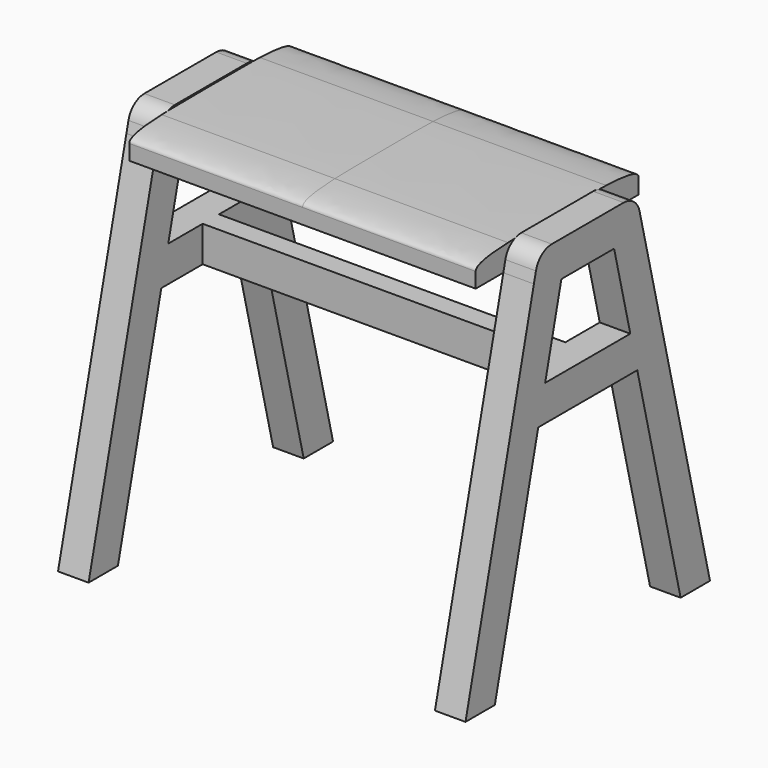
from build123d import *

# Parameters (mm, degrees)
F0_W        = 1
F0_H        = 3.5
F1_DEPTH    = 3
F2_DEPTH    = 20
F4_DEPTH    = 17
F6_T1_DEPTH = 6.9276237231
F6_T3_DEPTH = 6.9276237231


# Not quite as in the source:
# - a fillet or chamfer that OpenCascade refuses, or shapes differently, is made with other operations: its cross-section is extruded or revolved along the edge and cut away or added


with BuildPart() as f1:
    # F0 (on Right) → F1 (new body)
    with BuildSketch(Plane.YZ):
        Polygon((-185.4956659779, 34.4343371689), (-193.88920142, 0), (-190.2867229659, 0), (-184.9662980764, 21.8269531103), (-184.1131562284, 25.3269531103), (-182.1236807397, 33.4887426496), (-178.88920142, 33.4887426496), (-175.6547221004, 33.4887426496), (-173.6652466117, 25.3269531103), (-172.8121047636, 21.8269531103), (-167.4916798742, 0), (-163.88920142, 0), (-172.2827368621, 34.4343371689), (-178.88920142, 34.4343371689), align=None)
        Polygon((-184.8730173458, 36.9887426496), (-185.4956659779, 34.4343371689), (-178.88920142, 34.4343371689), (-172.2827368621, 34.4343371689), (-172.9053854942, 36.9887426496), (-178.88920142, 36.9887426496), align=None)
        Polygon((-184.1131562284, 25.3269531103), (-184.9662980764, 21.8269531103), (-179.88920142, 21.8269531103), (-179.88920142, 25.3269531103), align=None)
        with Locations((-178.38920142, 23.5769531103)):
            Rectangle(F0_W, F0_H)
        with Locations((-179.38920142, 23.5769531103)):
            Rectangle(F0_W, F0_H)
        Polygon((-177.88920142, 21.8269531103), (-172.8121047636, 21.8269531103), (-173.6652466117, 25.3269531103), (-177.88920142, 25.3269531103), align=None)
    extrude(amount=-F1_DEPTH)

    # F0 (on Right) → F2 (join)
    with BuildSketch(Plane.YZ):
        with Locations((-179.38920142, 23.5769531103)):
            Rectangle(F0_W, F0_H)
        with Locations((-178.38920142, 23.5769531103)):
            Rectangle(F0_W, F0_H)
    extrude(amount=-F2_DEPTH)

    # F3 (on face) → F4 (join, through all)
    with BuildSketch(Plane(origin=(-3, 0, 0), x_dir=(0, -1, 0), z_dir=(-1, 0, 0))):
        with BuildLine():
            Line((168.88920142, 34.4301523733), (172.2817167981, 34.4301523733))
            Line((172.2817167981, 34.4301523733), (172.8685340256, 36.8375601227))
            add(Edge.make_bspline(
                [(168.88920142, 35.9301523733), (168.88920142, 36.5362981599), (170.5285389627, 36.7602466997), (172.8685340256, 36.8375601227)],
                knots=[0, 0, 0, 0, 0.2862985804, 0.2862985804, 0.2862985804, 0.2862985804], degree=3))
            Line((168.88920142, 35.9301523733), (168.88920142, 34.4301523733))
        make_face()
        with BuildLine():
            Line((184.9191853663, 36.7993391266), (185.496686042, 34.4301523733))
            Line((185.496686042, 34.4301523733), (188.88920142, 34.4301523733))
            Line((188.88920142, 34.4301523733), (188.88920142, 35.9301523733))
            add(Edge.make_bspline(
                [(184.9191853663, 36.7993391266), (187.2542140028, 36.7124384565), (188.88920142, 36.4941599471), (188.88920142, 35.9301523733)],
                knots=[0.7140815311, 0.7140815311, 0.7140815311, 0.7140815311, 1, 1, 1, 1], degree=3))
        make_face()
        with BuildLine():
            Line((172.2817167981, 34.4301523733), (178.88920142, 34.4301523733))
            Line((178.88920142, 34.4301523733), (185.496686042, 34.4301523733))
            Line((185.496686042, 34.4301523733), (184.9191853663, 36.7993391266))
            add(Edge.make_bspline(
                [(172.8685340256, 36.8375601227), (174.6151730279, 36.895269065), (178.8930025349, 36.8472471546), (183.1708320419, 36.8644060269), (184.9191853663, 36.7993391266)],
                knots=[0.2862985804, 0.2862985804, 0.2862985804, 0.2862985804, 0.5, 0.7140815311, 0.7140815311, 0.7140815311, 0.7140815311], degree=3))
            Line((172.8685340256, 36.8375601227), (172.2817167981, 34.4301523733))
        make_face()
    extrude(amount=F4_DEPTH)

    # F5: F1 across face


with BuildPart() as f1_1:
    add(f1.part)
    add(f1.part.mirror(Plane(origin=(-20, -178.8538492179, 35.6039729667), x_dir=(0, -1, 0), z_dir=(-1, 0, 0))))

    # F6: fillet of radius 2 on 4 edges, made by hand

    # F6_s2 → F6_t1 (cut)
    with BuildSketch(Plane.YZ.offset(-3)):
        with BuildLine():
            ThreePointArc((-185.2450745508, 35.4623842598), (-184.5374266336, 36.561524138), (-183.3019678566, 36.9887426496))
            Line((-183.3019678566, 36.9887426496), (-184.8730173458, 36.9887426496))
            Line((-184.8730173458, 36.9887426496), (-185.2450745508, 35.4623842598))
        make_face()
        with BuildLine():
            ThreePointArc((-172.5333282893, 35.4623842598), (-173.2409762064, 36.561524138), (-174.4764349835, 36.9887426496))
            Line((-174.4764349835, 36.9887426496), (-172.9053854942, 36.9887426496))
            Line((-172.9053854942, 36.9887426496), (-172.5333282893, 35.4623842598))
        make_face()
    extrude(amount=F6_T1_DEPTH, mode=Mode.SUBTRACT)

    # F6_s4 → F6_t3 (cut)
    with BuildSketch(Plane.YZ.offset(-43.9276237231)):
        with BuildLine():
            ThreePointArc((-185.2450745508, 35.4623842598), (-184.5374266336, 36.561524138), (-183.3019678566, 36.9887426496))
            Line((-183.3019678566, 36.9887426496), (-184.8730173458, 36.9887426496))
            Line((-184.8730173458, 36.9887426496), (-185.2450745508, 35.4623842598))
        make_face()
        with BuildLine():
            ThreePointArc((-172.5333282893, 35.4623842598), (-173.2409762064, 36.561524138), (-174.4764349835, 36.9887426496))
            Line((-174.4764349835, 36.9887426496), (-172.9053854942, 36.9887426496))
            Line((-172.9053854942, 36.9887426496), (-172.5333282893, 35.4623842598))
        make_face()
    extrude(amount=F6_T3_DEPTH, mode=Mode.SUBTRACT)


solid = f1_1.part
